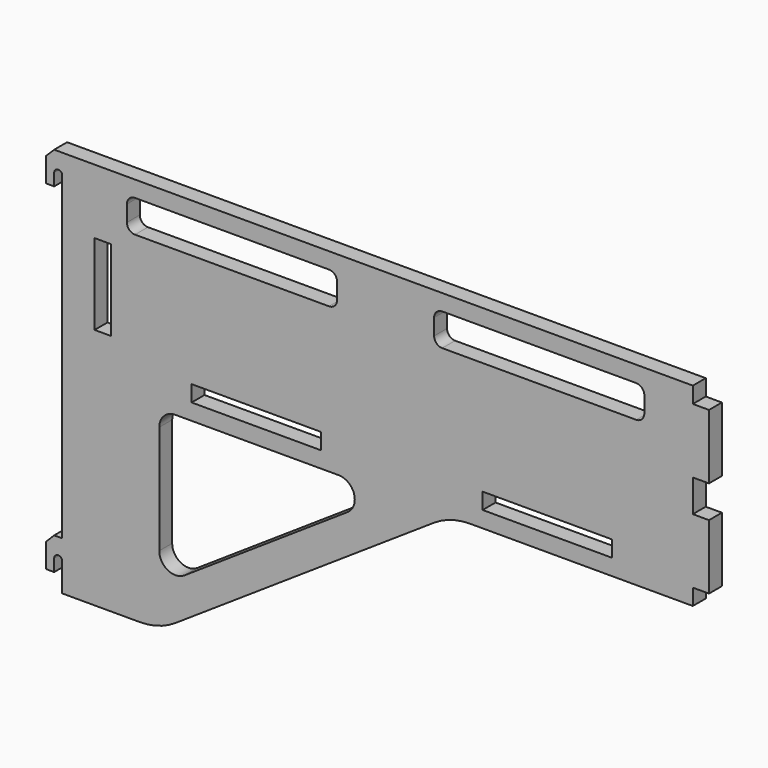
from build123d import *

# Parameters (mm, degrees)
F0_W     = 6.35
F0_H     = 31.75
F0_W_2   = 50.8
F0_H_2   = 6.35
F0_W_3   = 82.55
F0_H_3   = 12.7
F1_DEPTH = 6.35
F2_R     = 6.35
F3_R     = 25.4
F4_R     = 3.175
F6_DEPTH = 6.35
F7_R     = 1.58749
F8_SIZE  = 3.175


# Not quite as in the source:
# - a fillet or chamfer is up to 0.001 mm smaller than in the source, because OpenCascade refuses the exact size


with BuildPart() as f1:
    # F0 (on Front) → F1 (new body)
    with BuildSketch(Plane.XZ):
        Polygon((120.65, 76.2), (-127, 76.2), (-127, -76.2), (-88.9, -76.2), (25.4, 0), (120.65, 0), (120.65, 6.35), (127, 6.35), (127, 31.75), (120.65, 31.75), (120.65, 44.45), (127, 44.45), (127, 69.85), (120.65, 69.85), align=None)
        Polygon((2.5047494008, 0), (-88.9, -60.9364996005), (-88.9, 0), align=None, mode=Mode.SUBTRACT)
        with Locations((-111.125, 34.925)):
            Rectangle(F0_W, F0_H, mode=Mode.SUBTRACT)
        with Locations((-50.8, 9.525)):
            Rectangle(F0_W_2, F0_H_2, mode=Mode.SUBTRACT)
        with Locations((-60.325, 63.5)):
            Rectangle(F0_W_3, F0_H_3, mode=Mode.SUBTRACT)
        with Locations((63.5, 9.525)):
            Rectangle(F0_W_2, F0_H_2, mode=Mode.SUBTRACT)
        with Locations((60.325, 63.5)):
            Rectangle(F0_W_3, F0_H_3, mode=Mode.SUBTRACT)
    extrude(amount=F1_DEPTH)

    # F2
    f2_edges = [f1.edges().sort_by_distance(p)[0] for p in [
        (2.504749, -3.175, 0),
        (-88.9, -3.175, -60.9365),
        (-88.9, -3.175, 0),
    ]]
    fillet(f2_edges, radius=F2_R)

    # F3
    f3_edges = [f1.edges().sort_by_distance(p)[0] for p in [
        (25.4, -3.175, 0),
        (-88.9, -3.175, -76.2),
    ]]
    fillet(f3_edges, radius=F3_R)

    # F4
    f4_edges = [f1.edges().sort_by_distance(p)[0] for p in [
        (-101.6, -3.175, 57.15),
        (-101.6, -3.175, 69.85),
        (-19.05, -3.175, 57.15),
        (-19.05, -3.175, 69.85),
        (101.6, -3.175, 69.85),
        (101.6, -3.175, 57.15),
        (19.05, -3.175, 57.15),
        (19.05, -3.175, 69.85),
    ]]
    fillet(f4_edges, radius=F4_R)

    # F5 (on face) → F6 (join)
    with BuildSketch(Plane.XZ.offset(6.35)):
        Polygon((-127, 69.85), (-127, 76.2), (-133.35, 76.2), (-133.35, 63.5), (-130.175, 63.5), (-130.175, 69.85), align=None)
        Polygon((-130.175, -63.5), (-127, -63.5), (-127, -57.15), (-133.35, -57.15), (-133.35, -69.85), (-130.175, -69.85), align=None)
        Polygon((-127, -63.5), (-127, -57.15), (-133.35, -57.15), (-133.35, -69.85), (-130.175, -69.85), (-130.175, -63.5), align=None)
    extrude(amount=-F6_DEPTH)

    # F7 (radius 1.5875 in the source; OpenCascade refuses exactly that, so slightly less here)
    f7_edges = [f1.edges().sort_by_distance(p)[0] for p in [
        (-127, -3.175, 69.85),
        (-130.175, -3.175, 69.85),
        (-130.175, -3.175, -63.5),
        (-127, -3.175, -63.5),
    ]]
    fillet(f7_edges, radius=F7_R)

    # F8
    f8_edges = [f1.edges().sort_by_distance(p)[0] for p in [
        (-133.35, -3.175, 76.2),
        (-133.35, -3.175, -57.15),
    ]]
    chamfer(f8_edges, length=F8_SIZE)


solid = f1.part
